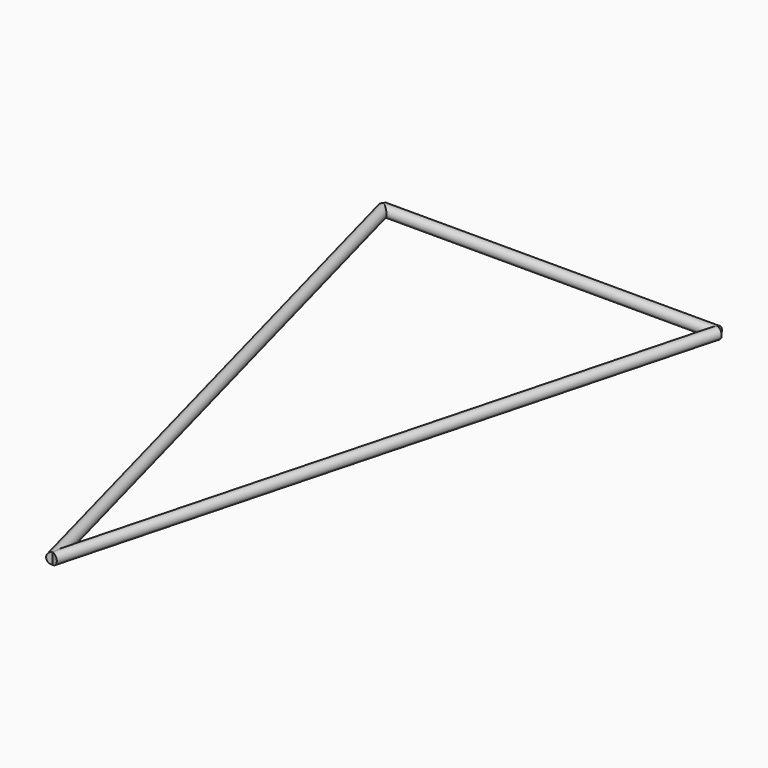
from build123d import *

# Parameters (mm, degrees)
F4_E2_W = 1524
F4_E2_H = 25.4
F3_E1_W = 2944.1419185291
F3_E1_H = 25.4


# Not quite as in the source:
# - a feature of the source that left no trace in its solid (it failed there, or was rolled back) is left out
# - a pattern or mirror of a feature is missing from the dataset's text; its kind, count and spacing are read off the source's solid


with BuildPart() as f5:
    # F4_E2 (on explicit) → F5 (revolve)
    with BuildSketch(Plane(origin=(-762, 1890.9206461344, 0), x_dir=(1, 0, 0), z_dir=(0, -1, 0))):
        with Locations((762, 12.7)):
            Rectangle(F4_E2_W, F4_E2_H)
    revolve(axis=Axis((0, 1890.9206461344, 0), (1, 0, 0)))

    # F3_E1 (on explicit) → F6 (revolve)
    with BuildSketch(Plane(origin=(0, -952.9020692331, 0), x_dir=(-0.2588190451, 0.9659258263, 0), z_dir=(0.9659258263, 0.2588190451, 0))):
        with Locations((1472.0709592645, 12.7)):
            Rectangle(F3_E1_W, F3_E1_H)
    f6 = revolve(axis=Axis((-381, 469.0092884507, 0), (-0.2588190451, 0.9659258263, 0)))

    # F6_copies: F6 across plane
    add(f6.mirror(Plane(origin=(0, 0, 0), x_dir=(0, 0, 1), z_dir=(1, 0, 0))))


solid = f5.part
